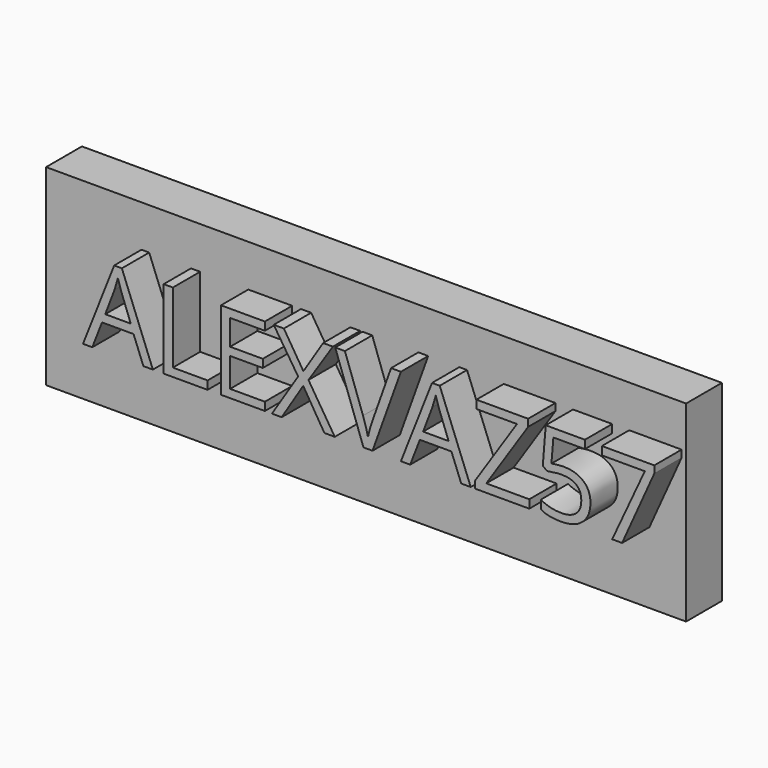
from build123d import *

# Parameters (mm, degrees)
F1_TEXT_SIZE = 13.1393799518
F2_DEPTH     = 4.064
F0_W         = 76.2
F0_H         = 22.86
F3_DEPTH     = 5.334


# Not quite as in the source:
# - Text() gives the source's letters only with a copy of the font that has no kerning and outlines rounded to 1/6400 em; it was checked with that copy


with BuildPart() as f2:
    # F1 (on face) → F2 (new body)
    with BuildSketch(Plane.XZ):
        with Locations((-34.4344141004, 8.4747146527)):
            Text('ALEXVAZ57', F1_TEXT_SIZE, font='Open Sans', text_align=(TextAlign.LEFT, TextAlign.BOTTOM))
    extrude(amount=F2_DEPTH)


with BuildPart() as f3:
    # F0 (on Front) → F3 (new body)
    with BuildSketch(Plane.XZ):
        with Locations((-3.9842394233, 11.43)):
            Rectangle(F0_W, F0_H)
    extrude(amount=-F3_DEPTH)


solid = Compound([f2.part, f3.part])
